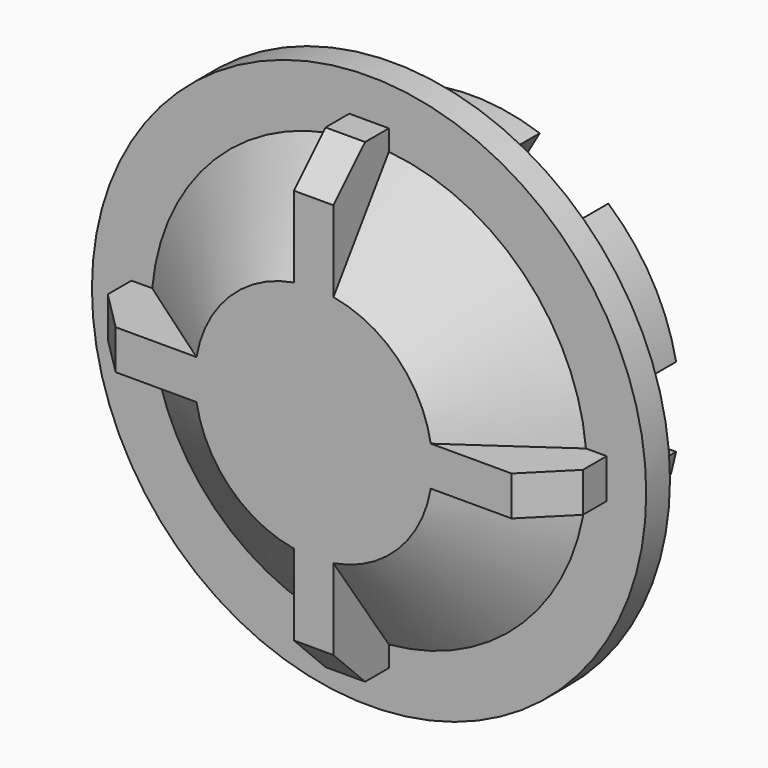
from build123d import *

# Parameters (mm, degrees)
F2_W     = 3.9979876956
F2_H     = 4
F3_DEPTH = 5
F4_W     = 8
F4_H     = 2
F4_W_2   = 2
F4_H_2   = 8
F5_DEPTH = 3.5
F6_SIZE  = 2


with BuildPart() as f1:
    # F0 (on Top) → F1 (revolve)
    with BuildSketch(Plane.XY):
        Polygon((0, 1.5), (0, 0), (6, 0), (11, 3.5), (14, 3.5), (14, 5), (10.5, 5), (10.5, 10), (9.3, 10), (9.3, 4.1409833424), (5.5271666538, 1.5), align=None)
    revolve(axis=Axis((0, 5.6900531054, 0), (0, 1, 0)))

    # F2 (on face) → F3 (cut, through all)
    with BuildSketch(Plane(origin=(0, 10, 0), x_dir=(-1, 0, 0), z_dir=(0, 1, 0))):
        with Locations((9.9453665316, 0)):
            Rectangle(F2_W, F2_H)
        Polygon((4.2401293821, 11.3441195205), (2.2411355343, 7.8817606121), (5.7052371495, 5.8817606121), (7.7042309973, 9.3441195205), align=None)
        Polygon((-7.7042309973, 9.3441195205), (-5.7052371495, 5.8817606121), (-2.2411355343, 7.8817606121), (-4.2401293821, 11.3441195205), align=None)
        with Locations((-9.9453665316, 0)):
            Rectangle(F2_W, F2_H)
        Polygon((-4.2401293821, -11.3441195205), (-2.2411355343, -7.8817606121), (-5.7052371495, -5.8817606121), (-7.7042309973, -9.3441195205), align=None)
        Polygon((7.7042309973, -9.3441195205), (5.7052371495, -5.8817606121), (2.2411355343, -7.8817606121), (4.2401293821, -11.3441195205), align=None)
    extrude(amount=-F3_DEPTH, mode=Mode.SUBTRACT)

    # F4 (on face) → F5 (join, through all)
    with BuildSketch(Plane.XZ):
        with Locations((-8, 0)):
            Rectangle(F4_W, F4_H)
        with Locations((0, -8)):
            Rectangle(F4_W_2, F4_H_2)
        with Locations((8, 0)):
            Rectangle(F4_W, F4_H)
        with Locations((0, 8)):
            Rectangle(F4_W_2, F4_H_2)
    extrude(amount=-F5_DEPTH)

    # F6
    f6_edges = [f1.edges().sort_by_distance(p)[0] for p in [
        (-12, 0, 0),
        (0, 0, -12),
        (12, 0, 0),
        (0, 0, 12),
    ]]
    chamfer(f6_edges, length=F6_SIZE)


solid = f1.part
